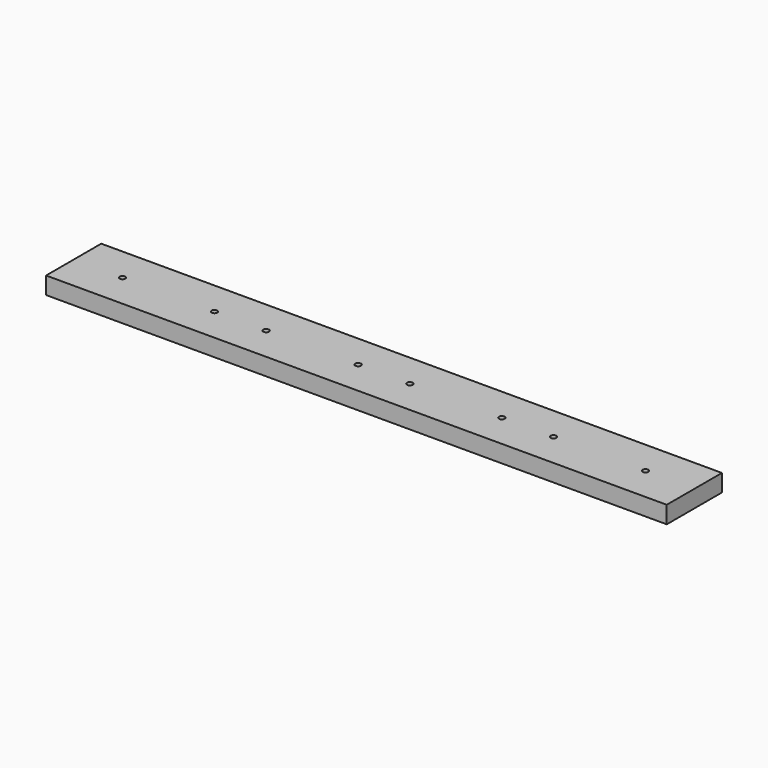
from build123d import *

# Parameters (mm, degrees)
F1_W     = 685.8
F1_H     = 76.2
F1_R     = 3.175
F2_DEPTH = 19.05


# Not quite as in the source:
# - a variable given as a bare number and used for a length is read in inches; the dataset says mm whatever the document's units were


with BuildPart() as f2:
    # F1 (on Top) → F2 (new body)
    with BuildSketch(Plane.XY):
        Rectangle(F1_W, F1_H)
        with Locations((-288.925, 0)):
            Circle(F1_R, mode=Mode.SUBTRACT)
        with Locations((-187.325, 0)):
            Circle(F1_R, mode=Mode.SUBTRACT)
        with Locations((-130.175, 0)):
            Circle(F1_R, mode=Mode.SUBTRACT)
        with Locations((-28.575, 0)):
            Circle(F1_R, mode=Mode.SUBTRACT)
        with Locations((28.575, 0)):
            Circle(F1_R, mode=Mode.SUBTRACT)
        with Locations((130.175, 0)):
            Circle(F1_R, mode=Mode.SUBTRACT)
        with Locations((187.325, 0)):
            Circle(F1_R, mode=Mode.SUBTRACT)
        with Locations((288.925, 0)):
            Circle(F1_R, mode=Mode.SUBTRACT)
    extrude(amount=F2_DEPTH)


solid = f2.part
